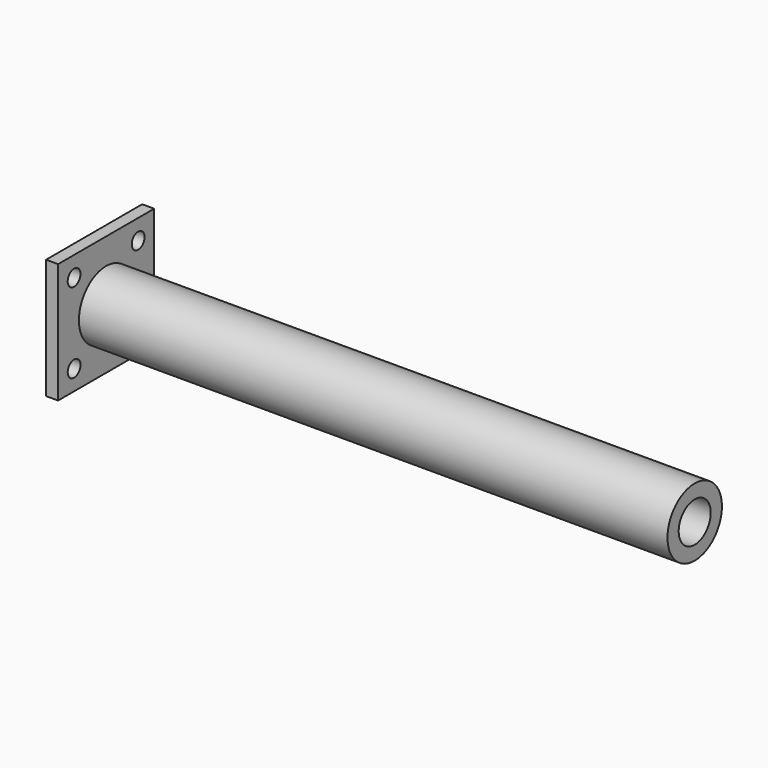
from build123d import *
from build123d import SkipClean  # not in build123d's __all__

# Parameters (mm, degrees)
F0_R      = 8.5
F0_R_2    = 7
F1_DEPTH  = 150
F2_R      = 7
F2_R_2    = 5
F3_DEPTH  = 145
F4_W      = 30
F4_H      = 30
F4_R      = 8.5
F5_DEPTH  = 3
F7_D      = 4
F9_DEPTH  = 140
F12_ANGLE = 90
F14_DEPTH = 5
F15_W     = 2.5
F15_H     = 2.0939723571
F16_ANGLE = 90
F18_DEPTH = 10
F19_W     = 5
F19_H     = 2.0680303106
F20_ANGLE = 90
F22_DEPTH = 5
F23_W     = 5
F23_H     = 2.0939723571
F24_ANGLE = 90
F26_DEPTH = 10
F27_W     = 5
F27_H     = 2.0939723571
F28_ANGLE = 90
F30_DEPTH = 5


# Not quite as in the source:
# - after a boolean that leaves OpenCascade's solid faulty, fix() repairs it


with BuildPart() as f1:
    # F0 (on Right) → F1 (new body)
    with BuildSketch(Plane.YZ):
        Circle(F0_R)
        Circle(F0_R_2, mode=Mode.SUBTRACT)
    extrude(amount=F1_DEPTH)

    # F2 (on face) → F3 (join)
    with BuildSketch(Plane.YZ.offset(150)):
        Circle(F2_R)
        Circle(F2_R_2, mode=Mode.SUBTRACT)
    extrude(amount=-F3_DEPTH)

    # F4 (on face) → F5 (join)
    with BuildSketch(Plane(origin=(0, 0, 0), x_dir=(0, -1, 0), z_dir=(-1, 0, 0))):
        Rectangle(F4_W, F4_H)
        Circle(F4_R, mode=Mode.SUBTRACT)
    extrude(amount=-F5_DEPTH)

    # F7 (through all)
    with Locations(Plane(origin=(0, 0, 0), x_dir=(0, -1, 0), z_dir=(-1, 0, 0))):
        with Locations((-10, 10), (10, 10), (10, -10), (-10, -10)):
            Hole(F7_D / 2)

    # F8 (on face) → F9 (cut)
    with BuildSketch(Plane(origin=(5, 0, 0), x_dir=(0, -1, 0), z_dir=(-1, 0, 0))):
        with BuildLine():
            ThreePointArc((0, 5), (0.8891730726, 4.9203019467), (1.75, 4.6837484988))
            Line((1.75, 4.6837484988), (1.75, 6.7777208559))
            ThreePointArc((1.75, 6.7777208559), (0.8820300474, 6.9442078739), (0, 7))
            Line((0, 7), (0, 5))
        make_face()
        with BuildLine():
            ThreePointArc((-1.75, 4.6837484988), (-0.8891730726, 4.9203019467), (0, 5))
            Line((0, 5), (0, 7))
            ThreePointArc((0, 7), (-0.8820300474, 6.9442078739), (-1.75, 6.7777208559))
            Line((-1.75, 6.7777208559), (-1.75, 4.6837484988))
        make_face()
    extrude(amount=-F9_DEPTH, mode=Mode.SUBTRACT)

    # F10 (on face) → F12 (revolve, cut)
    with BuildSketch(Plane(origin=(0, -1.75, 0), x_dir=(-1, 0, 0), z_dir=(0, 1, 0))):
        Polygon((-140, 6.7777208559), (-140, 4.7096905453), (-140, 4.6837484988), (-135, 4.6837484988), (-135, 6.7777208559), align=None)
    revolve(axis=Axis((74.9857723713, 0, 0), (1, 0, 0)), revolution_arc=F12_ANGLE, mode=Mode.SUBTRACT)

    # F13 (on face) → F14 (cut)
    with BuildSketch(Plane(origin=(140, 0, 0), x_dir=(0, -1, 0), z_dir=(-1, 0, 0))):
        with BuildLine():
            Line((6.0300092452, 3.5551355111), (4.5493471919, 2.0744734578))
            ThreePointArc((4.5493471919, 2.0744734578), (4.9969153801, 0.17560377), (4.6837484988, -1.75))
            Line((4.6837484988, -1.75), (6.7777208559, -1.75))
            ThreePointArc((6.7777208559, -1.75), (6.9314935824, 0.9769322988), (6.0300092452, 3.5551355111))
        make_face()
    with SkipClean():  # cleaning this boolean's faces spoils the solid; the shape is the same uncleaned
        extrude(amount=-F14_DEPTH, mode=Mode.SUBTRACT)

    # F15 (on face) → F16 (revolve, cut)
    with BuildSketch(Plane(origin=(0, -1.75, 0), x_dir=(-1, 0, 0), z_dir=(0, 1, 0))):
        with Locations((-68.75, 5.7307346773)):
            Rectangle(F15_W, F15_H)
        with Locations((-71.25, 5.7307346773)):
            Rectangle(F15_W, F15_H)
    revolve(axis=Axis((74.9857723713, 0, 0), (1, 0, 0)), revolution_arc=F16_ANGLE, mode=Mode.SUBTRACT)

    add(f1.part.fix(), mode=Mode.REPLACE)

    # F17 (on face) → F18 (cut)
    with BuildSketch(Plane.YZ.offset(67.5)):
        with BuildLine():
            ThreePointArc((-4.6837484988, -1.75), (-4.9969153801, 0.17560377), (-4.5493471919, 2.0744734578))
            Line((-4.5493471919, 2.0744734578), (-6.0300092452, 3.5551355111))
            ThreePointArc((-6.0300092452, 3.5551355111), (-6.9314935824, 0.9769322988), (-6.7777208559, -1.75))
            Line((-6.7777208559, -1.75), (-4.6837484988, -1.75))
        make_face()
    extrude(amount=F18_DEPTH, mode=Mode.SUBTRACT)

    # F19 (on face) → F20 (revolve, cut)
    with BuildSketch(Plane(origin=(0, -1.75, 0), x_dir=(-1, 0, 0), z_dir=(0, 1, 0))):
        with Locations((-109.95097965, 5.8026228816)):
            Rectangle(F19_W, F19_H)
    revolve(axis=Axis((112.4786585569, 0, 0), (1, 0, 0)), revolution_arc=F20_ANGLE, mode=Mode.SUBTRACT)

    # F21 (on face) → F22 (cut)
    with BuildSketch(Plane(origin=(112.45097965, 0, 0), x_dir=(0, -1, 0), z_dir=(-1, 0, 0))):
        with BuildLine():
            ThreePointArc((6.8366380369, -1.75), (6.9854372426, 1.0028889159), (6.068155613, 3.6027221796))
            Line((6.068155613, 3.6027221796), (4.6366684016, 2.07447))
            ThreePointArc((4.6366684016, 2.07447), (5.0765586233, 0.1751347812), (4.7686077263, -1.75))
            Line((4.7686077263, -1.75), (6.8366380369, -1.75))
        make_face()
    extrude(amount=-F22_DEPTH, mode=Mode.SUBTRACT)

    # F23 (on face) → F24 (revolve, cut)
    with BuildSketch(Plane(origin=(0, -1.75, 0), x_dir=(-1, 0, 0), z_dir=(0, 1, 0))):
        with Locations((-33.75, 5.7307346773)):
            Rectangle(F23_W, F23_H)
    revolve(axis=Axis((74.9857723713, 0, 0), (1, 0, 0)), revolution_arc=F24_ANGLE, mode=Mode.SUBTRACT)

    # F25 (on face) → F26 (cut)
    with BuildSketch(Plane.YZ.offset(31.25)):
        with BuildLine():
            ThreePointArc((-4.6837484988, -1.75), (-4.9969153801, 0.17560377), (-4.5493471919, 2.0744734578))
            Line((-4.5493471919, 2.0744734578), (-6.0300092452, 3.5551355111))
            ThreePointArc((-6.0300092452, 3.5551355111), (-6.9314935824, 0.9769322988), (-6.7777208559, -1.75))
            Line((-6.7777208559, -1.75), (-4.6837484988, -1.75))
        make_face()
    extrude(amount=F26_DEPTH, mode=Mode.SUBTRACT)

    # F27 (on face) → F28 (revolve)
    with BuildSketch(Plane(origin=(0, -1.75, 0), x_dir=(-1, 0, 0), z_dir=(0, 1, 0))):
        with Locations((-7.5, 5.7307346773)):
            Rectangle(F27_W, F27_H)
    revolve(axis=Axis((74.9857723713, 0, 0), (1, 0, 0)), revolution_arc=F28_ANGLE)

    # F29 (on face) → F30 (cut)
    with BuildSketch(Plane(origin=(5, 0, 0), x_dir=(0, -1, 0), z_dir=(-1, 0, 0))):
        with BuildLine():
            Line((5.896972825, 3.7716987554), (4.4710360492, 2.2382664379))
            ThreePointArc((4.4710360492, 2.2382664379), (4.9875229666, 0.3530080143), (4.7417252408, -1.5862035621))
            Line((4.7417252408, -1.5862035621), (6.8179145096, -1.5862035621))
            ThreePointArc((6.8179145096, -1.5862035621), (6.8988310092, 1.185803823), (5.896972825, 3.7716987554))
        make_face()
    extrude(amount=-F30_DEPTH, mode=Mode.SUBTRACT)

    add(f1.part.fix(), mode=Mode.REPLACE)


solid = f1.part
